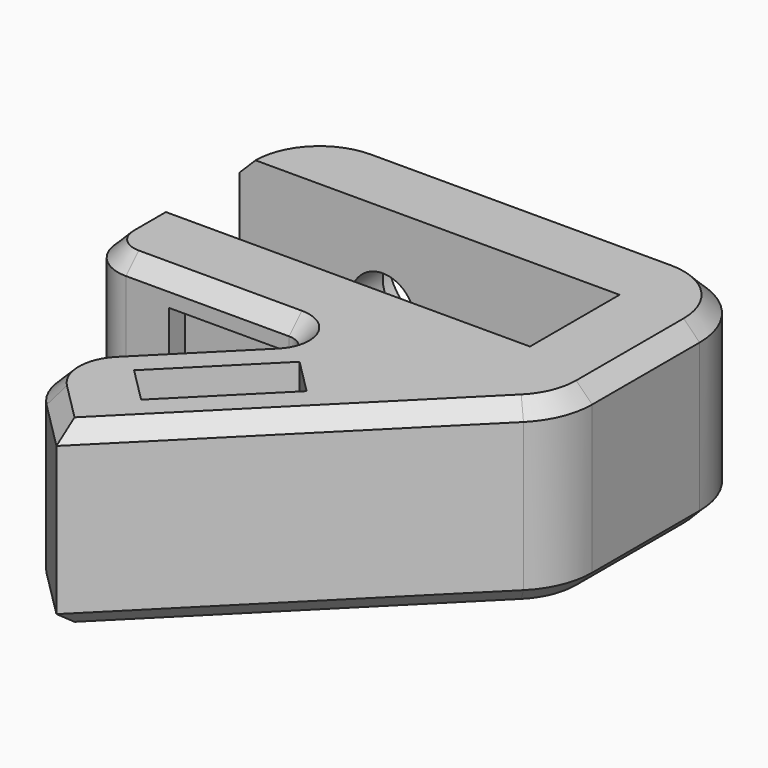
from build123d import *

# Parameters (mm, degrees)
F1_DEPTH      = 9
F2_R          = 3.99999
F3_R          = 1
F4_R          = 2
F5_W          = 6
F5_H          = 6
F6_DEPTH      = 1
F7_R          = 1.6
F8_DEPTH      = 12.601
F9_R          = 3
F9_R_2        = 1.6
F10_DEPTH     = 2
F12_DEPTH     = 9.001
F13_R         = 3
F14_T1_DEPTH  = 20.400496283
F14_T3_DEPTH  = 8.1624490891
F14_T5_DEPTH  = 15.00002
F14_T7_DEPTH  = 6.3449613941
F14_T9_DEPTH  = 5.5573463904
F14_T11_DEPTH = 4.0573463904
F14_T13_DEPTH = 2.0573563904
F14_T15_DEPTH = 6.7122106995
F14_T18_ANGLE = 90
F14_T20_ANGLE = 135
F14_T22_ANGLE = 90
F14_T24_ANGLE = 90
F14_T26_ANGLE = 90
F14_T28_ANGLE = 45
F14_T30_ANGLE = 90
F14_T32_ANGLE = 135
F14_T34_ANGLE = 90
F14_T36_ANGLE = 45
F14_T38_ANGLE = 90
F14_T40_ANGLE = 90


# Not quite as in the source:
# - a fillet or chamfer that OpenCascade refuses, or shapes differently, is made with other operations: its cross-section is extruded or revolved along the edge and cut away or added
# - a fillet or chamfer is up to 0.001 mm smaller than in the source, because OpenCascade refuses the exact size


with BuildPart() as f1:
    # F0 (on Top) → F1 (new body)
    with BuildSketch(Plane.XY):
        Polygon((0, 4), (0, 0), (12.5766626515, 0), (4.2616702986, -8.3149923529), (8.8578643763, -12.9111864306), (23, 1.2309491931), (23, 13.6), (0, 13.6), (0, 9.6), (19, 9.6), (19, 4), align=None)
    extrude(amount=F1_DEPTH)

    # F2 (radius 4 in the source; OpenCascade refuses exactly that, so slightly less here)
    f2_edges = [f1.edges().sort_by_distance(p)[0] for p in [
        (23, 13.6, 4.5),
        (0, 13.6, 4.5),
        (23, 1.230949, 4.5),
    ]]
    fillet(f2_edges, radius=F2_R)

    # F3
    f3_edges = [f1.edges().sort_by_distance(p)[0] for p in [
        (12.576663, 0, 4.5),
    ]]
    fillet(f3_edges, radius=F3_R)

    # F4
    f4_edges = [f1.edges().sort_by_distance(p)[0] for p in [
        (0, 0, 4.5),
    ]]
    fillet(f4_edges, radius=F4_R)

    # F5 (on face) → F6 (cut)
    with BuildSketch(Plane.XZ):
        with Locations((7.1624490891, 4.5)):
            Rectangle(F5_W, F5_H)
    extrude(amount=-F6_DEPTH, mode=Mode.SUBTRACT)

    # F7 (on face) → F8 (cut, through all)
    with BuildSketch(Plane.XZ.offset(-1)):
        with Locations((7.1624490891, 4.5)):
            Circle(F7_R)
    extrude(amount=-F8_DEPTH, mode=Mode.SUBTRACT)

    # F9 (on face) → F10 (cut)
    with BuildSketch(Plane(origin=(0, 13.6, 0), x_dir=(-1, 0, 0), z_dir=(0, 1, 0))):
        with Locations((-7.1624490891, 4.5)):
            Circle(F9_R)
        with Locations((-7.1624490891, 4.5)):
            Circle(F9_R_2, mode=Mode.SUBTRACT)
    extrude(amount=-F10_DEPTH, mode=Mode.SUBTRACT)

    # F11 (on face) → F12 (cut, through all)
    with BuildSketch(Plane(origin=(0, 0, 0), x_dir=(1, 0, 0), z_dir=(0, 0, -1))):
        Polygon((12.7809664736, 2.6241233026), (14.5487334265, 4.3918902556), (9.9525393488, 8.9880843333), (8.1847723959, 7.2203173803), align=None)
    extrude(amount=-F12_DEPTH, mode=Mode.SUBTRACT)

    # F13
    f13_edges = [f1.edges().sort_by_distance(p)[0] for p in [
        (4.26167, -8.314992, 4.5),
    ]]
    fillet(f13_edges, radius=F13_R)

    # F14: chamfer of 0.8 on 4 edges, made by hand

    # F14_s2 → F14_t1 (cut)
    with BuildSketch(Plane(origin=(-3.4814246111, -3.4814246111, 0), x_dir=(0, 0, 1), z_dir=(0.7071067812, 0.7071067812, 0))):
        Polygon((8.2, 15.3930434455), (9, 14.5930434455), (9, 15.3930434455), align=None)
        Polygon((0, 14.5930434455), (0.8, 15.3930434455), (0, 15.3930434455), align=None)
    extrude(amount=F14_T1_DEPTH, mode=Mode.SUBTRACT)

    # F14_s4 → F14_t3 (cut)
    with BuildSketch(Plane.YZ.offset(2)):
        Polygon((0, 8.2), (0.8, 9), (0, 9), align=None)
        Polygon((0.8, 0), (0, 0.8), (0, 0), align=None)
    extrude(amount=F14_T3_DEPTH, mode=Mode.SUBTRACT)

    # F14_s6 → F14_t5 (cut)
    with BuildSketch(Plane.YZ.offset(3.99999)):
        Polygon((12.8, 0), (13.6, 0.8), (13.6, 0), align=None)
        Polygon((13.6, 8.2), (12.8, 9), (13.6, 9), align=None)
    extrude(amount=F14_T5_DEPTH, mode=Mode.SUBTRACT)

    # F14_s8 → F14_t7 (cut)
    with BuildSketch(Plane(origin=(4.5812245445, 4.5812245445, 0), x_dir=(0, 0, 1), z_dir=(-0.7071067812, -0.7071067812, 0))):
        Polygon((0, -9.6930434455), (0.8, -8.8930434455), (0, -8.8930434455), align=None)
        Polygon((8.2, -8.8930434455), (9, -9.6930434455), (9, -8.8930434455), align=None)
    extrude(amount=F14_T7_DEPTH, mode=Mode.SUBTRACT)

    # F14_s10 → F14_t9 (cut)
    with BuildSketch(Plane(origin=(8.4096516693, -8.4096516693, 0), x_dir=(0, 0, 1), z_dir=(0.7071067812, -0.7071067812, 0))):
        Polygon((0, 2.066131511), (0.8, 2.866131511), (0, 2.866131511), align=None)
        Polygon((8.2, 2.866131511), (9, 2.066131511), (9, 2.866131511), align=None)
    extrude(amount=F14_T9_DEPTH, mode=Mode.SUBTRACT)

    # F14_s12 → F14_t11 (cut)
    with BuildSketch(Plane.XZ.offset(-6.0573463904)):
        Polygon((0.8, 0), (0, 0.8), (0, 0), align=None)
        Polygon((0, 8.2), (0.8, 9), (0, 9), align=None)
    extrude(amount=F14_T11_DEPTH, mode=Mode.SUBTRACT)

    # F14_s14 → F14_t13 (cut)
    with BuildSketch(Plane.XZ.offset(-9.60001)):
        Polygon((0.8, 0), (0, 0.8), (0, 0), align=None)
        Polygon((0, 8.2), (0.8, 9), (0, 9), align=None)
    extrude(amount=F14_T13_DEPTH, mode=Mode.SUBTRACT)

    # F14_s16 → F14_t15 (cut)
    with BuildSketch(Plane.XZ.offset(-9.60001)):
        Polygon((22.2, 0), (23, 0.8), (23, 0), align=None)
        Polygon((23, 8.2), (22.2, 9), (23, 9), align=None)
    extrude(amount=F14_T15_DEPTH, mode=Mode.SUBTRACT)

    # F14_s17 → F14_t18 (revolve, cut)
    with BuildSketch(Plane.YZ.offset(2)):
        Polygon((0.8, 0), (0, 0.8), (0, 0), align=None)
    revolve(axis=Axis((2, 2, 0), (0, 0, -1)), revolution_arc=F14_T18_ANGLE, mode=Mode.SUBTRACT)

    # F14_s19 → F14_t20 (revolve, cut)
    with BuildSketch(Plane(origin=(4.5812245445, 4.5812245445, 0), x_dir=(0, 0, 1), z_dir=(-0.7071067812, -0.7071067812, 0))):
        Polygon((0, -9.6930434455), (0.8, -8.8930434455), (0, -8.8930434455), align=None)
    revolve(axis=Axis((10.1624490891, -1, 0), (0, 0, 1)), revolution_arc=F14_T20_ANGLE, mode=Mode.SUBTRACT)

    # F14_s21 → F14_t22 (revolve, cut)
    with BuildSketch(Plane(origin=(0.0946593164, 0.0946593164, 0), x_dir=(0, 0, 1), z_dir=(0.7071067812, 0.7071067812, 0))):
        Polygon((0, 9.6930434455), (0.8, 8.8930434455), (0, 8.8930434455), align=None)
    revolve(axis=Axis((8.5043109857, -8.3149923529, 0), (0, 0, 1)), revolution_arc=F14_T22_ANGLE, mode=Mode.SUBTRACT)

    # F14_s23 → F14_t24 (revolve, cut)
    with BuildSketch(Plane.XZ.offset(-9.60001)):
        Polygon((22.2, 0), (23, 0.8), (23, 0), align=None)
    revolve(axis=Axis((19.00001, 9.60001, 0), (0, 0, 1)), revolution_arc=F14_T24_ANGLE, mode=Mode.SUBTRACT)

    # F14_s25 → F14_t26 (revolve, cut)
    with BuildSketch(Plane.YZ.offset(3.99999)):
        Polygon((12.8, 0), (13.6, 0.8), (13.6, 0), align=None)
    revolve(axis=Axis((3.99999, 9.60001, 0), (0, 0, 1)), revolution_arc=F14_T26_ANGLE, mode=Mode.SUBTRACT)

    # F14_s27 → F14_t28 (revolve, cut)
    with BuildSketch(Plane(origin=(10.9439046502, 10.9439046502, 0), x_dir=(0, 0, 1), z_dir=(-0.7071067812, -0.7071067812, 0))):
        Polygon((0, -14.5930434455), (0.8, -15.3930434455), (0, -15.3930434455), align=None)
    revolve(axis=Axis((19.00001, 2.8877993005, 0), (0, 0, 1)), revolution_arc=F14_T28_ANGLE, mode=Mode.SUBTRACT)

    # F14_s29 → F14_t30 (revolve, cut)
    with BuildSketch(Plane.YZ.offset(2)):
        Polygon((0, 8.2), (0.8, 9), (0, 9), align=None)
    revolve(axis=Axis((2, 2, 9), (0, 0, -1)), revolution_arc=F14_T30_ANGLE, mode=Mode.SUBTRACT)

    # F14_s31 → F14_t32 (revolve, cut)
    with BuildSketch(Plane(origin=(4.5812245445, 4.5812245445, 0), x_dir=(0, 0, 1), z_dir=(-0.7071067812, -0.7071067812, 0))):
        Polygon((8.2, -8.8930434455), (9, -9.6930434455), (9, -8.8930434455), align=None)
    revolve(axis=Axis((10.1624490891, -1, 9), (0, 0, 1)), revolution_arc=F14_T32_ANGLE, mode=Mode.SUBTRACT)

    # F14_s33 → F14_t34 (revolve, cut)
    with BuildSketch(Plane(origin=(0.0946593164, 0.0946593164, 0), x_dir=(0, 0, 1), z_dir=(0.7071067812, 0.7071067812, 0))):
        Polygon((8.2, 8.8930434455), (9, 9.6930434455), (9, 8.8930434455), align=None)
    revolve(axis=Axis((8.5043109857, -8.3149923529, 9), (0, 0, 1)), revolution_arc=F14_T34_ANGLE, mode=Mode.SUBTRACT)

    # F14_s35 → F14_t36 (revolve, cut)
    with BuildSketch(Plane(origin=(10.9439046502, 10.9439046502, 0), x_dir=(0, 0, 1), z_dir=(-0.7071067812, -0.7071067812, 0))):
        Polygon((8.2, -15.3930434455), (9, -14.5930434455), (9, -15.3930434455), align=None)
    revolve(axis=Axis((19.00001, 2.8877993005, 9), (0, 0, 1)), revolution_arc=F14_T36_ANGLE, mode=Mode.SUBTRACT)

    # F14_s37 → F14_t38 (revolve, cut)
    with BuildSketch(Plane.XZ.offset(-9.60001)):
        Polygon((23, 8.2), (22.2, 9), (23, 9), align=None)
    revolve(axis=Axis((19.00001, 9.60001, 9), (0, 0, 1)), revolution_arc=F14_T38_ANGLE, mode=Mode.SUBTRACT)

    # F14_s39 → F14_t40 (revolve, cut)
    with BuildSketch(Plane.YZ.offset(3.99999)):
        Polygon((13.6, 8.2), (12.8, 9), (13.6, 9), align=None)
    revolve(axis=Axis((3.99999, 9.60001, 9), (0, 0, 1)), revolution_arc=F14_T40_ANGLE, mode=Mode.SUBTRACT)


solid = f1.part
